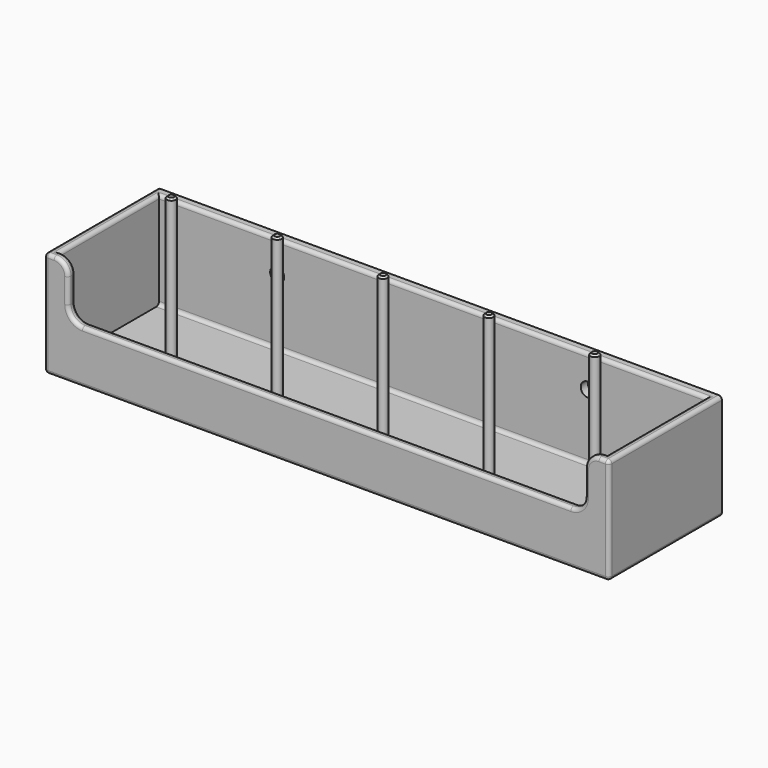
from build123d import *

# Parameters (mm, degrees)
F0_W      = 203.2
F0_H      = 38.1
F1_DEPTH  = 25.4
F2_W      = 196.85
F2_H      = 44.45
F3_DEPTH  = 34.925
F4_R      = 1.5875
F5_DEPTH  = 50.8
F6_W      = 185.9018951654
F6_H      = 9.962297976
F7_DEPTH  = 19.05
F8_R      = 5.08
F9_SIZE   = 0.635
F10_R     = 1.27
F11_R     = 2.54
F12_DEPTH = 5.08


with BuildPart() as f1:
    # F0 (on Front) → F1 (new body, symmetric)
    with BuildSketch(Plane.XZ):
        Rectangle(F0_W, F0_H)
    extrude(amount=F1_DEPTH, both=True)

    # F2 (on face) → F3 (cut)
    with BuildSketch(Plane.XY.offset(19.05)):
        Rectangle(F2_W, F2_H)
    extrude(amount=-F3_DEPTH, mode=Mode.SUBTRACT)

    # F4 (on face) → F5 (join)
    with BuildSketch(Plane.XY.offset(-15.875)):
        Circle(F4_R)
        with Locations((-38.1, 0)):
            Circle(F4_R)
        with Locations((-76.2, 0)):
            Circle(F4_R)
        with Locations((38.1, 0)):
            Circle(F4_R)
        with Locations((76.2, 0)):
            Circle(F4_R)
    extrude(amount=F5_DEPTH)

    # F6 (on face) → F7 (cut)
    with BuildSketch(Plane.XY.offset(19.05)):
        with Locations((0, -23.8689258695)):
            Rectangle(F6_W, F6_H)
    extrude(amount=-F7_DEPTH, mode=Mode.SUBTRACT)

    # F8
    f8_edges = [f1.edges().sort_by_distance(p)[0] for p in [
        (-92.950948, -23.8125, 19.05),
        (-92.950948, -23.8125, 0),
        (92.950948, -23.8125, 19.05),
        (92.950948, -23.8125, 0),
    ]]
    fillet(f8_edges, radius=F8_R)

    # F9
    f9_edges = [f1.edges().sort_by_distance(p)[0] for p in [
        (-1.5875, 0, 34.925),
        (-39.6875, 0, 34.925),
        (36.5125, 0, 34.925),
        (74.6125, 0, 34.925),
        (-77.7875, 0, 34.925),
    ]]
    chamfer(f9_edges, length=F9_SIZE)

    # F10
    f10_edges = [f1.edges().sort_by_distance(p)[0] for p in [
        (0, 22.225, 19.05),
        (-98.425, 0, 19.05),
        (0, -25.4, 0),
        (-91.46305, -25.4, 1.487898),
        (-92.950948, -25.4, 9.525),
        (-99.815474, -25.4, 19.05),
        (-101.6, 0, 19.05),
        (101.6, 0, 19.05),
        (101.6, -25.4, 0),
        (0, -25.4, -19.05),
        (101.6, 0, -19.05),
        (-101.6, -25.4, 0),
        (-101.6, 0, -19.05),
        (0, 22.225, -15.875),
        (0, -22.225, 0),
        (98.425, 0, 19.05),
        (98.425, 0, -15.875),
    ]]
    fillet(f10_edges, radius=F10_R)

    # F11 (on face) → F12 (cut)
    with BuildSketch(Plane.XZ.offset(-22.225)):
        with Locations((55.88, 7.5767044909)):
            Circle(F11_R)
        with Locations((-55.88, 7.5767044909)):
            Circle(F11_R)
    extrude(amount=-F12_DEPTH, mode=Mode.SUBTRACT)


solid = f1.part
